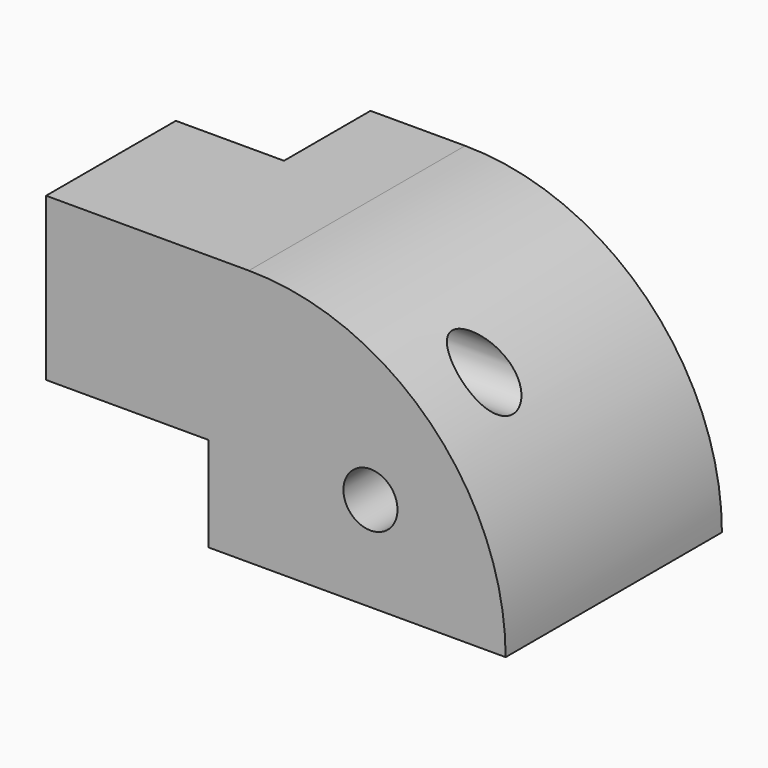
from build123d import *

# Parameters (mm, degrees)
F1_DEPTH  = 127
F2_DEPTH  = 127
F3_D      = 25.4
F0_W      = 76.2
F0_H      = 76.2
F4_DEPTH  = 76.2
F6_D      = 25.4
F9_W      = 50.8
F9_H      = 76.2
F10_DEPTH = 25.4


# Not quite as in the source:
# - a feature of the source that left no trace in its solid (it failed there, or was rolled back) is left out
# - a feature names something its author has since deleted; it is built from what else it names


with BuildPart() as f1:
    # F0 (on Front) → F1 (new body)
    with BuildSketch(Plane.XZ):
        with BuildLine():
            Line((0, 0), (120.65, 0))
            ThreePointArc((120.65, 0), (85.3124331502, 85.3124331502), (0, 120.65))
            Line((0, 120.65), (0, 44.45))
            Line((0, 44.45), (0, 0))
        make_face()
    extrude(amount=-F1_DEPTH)

    # F0 (on Front) → F2 (join)
    with BuildSketch(Plane.XZ):
        Polygon((0, 44.45), (0, 120.65), (-19.05, 120.65), (-19.05, 44.45), (-19.05, 0), (0, 0), align=None)
    extrude(amount=-F2_DEPTH)

    # F3 (through all)
    with Locations(Plane.XZ):
        with Locations((57.15, 44.45)):
            Hole(F3_D / 2)

    # F0 (on Front) → F4 (join)
    with BuildSketch(Plane.XZ):
        with Locations((-57.15, 82.55)):
            Rectangle(F0_W, F0_H)
    extrude(amount=-F4_DEPTH)

    # F6 (through all)
    with Locations(Plane(origin=(-95.25, 0, 0), x_dir=(0, -1, 0), z_dir=(-1, 0, 0))):
        with Locations((-38.1, 88.9)):
            Hole(F6_D / 2)

    # F9 (on face) → F10 (join)
    with BuildSketch(Plane(origin=(-19.05, 0, 0), x_dir=(0, -1, 0), z_dir=(-1, 0, 0))):
        with Locations((-101.6, 82.55)):
            Rectangle(F9_W, F9_H)
    extrude(amount=F10_DEPTH)


solid = f1.part
